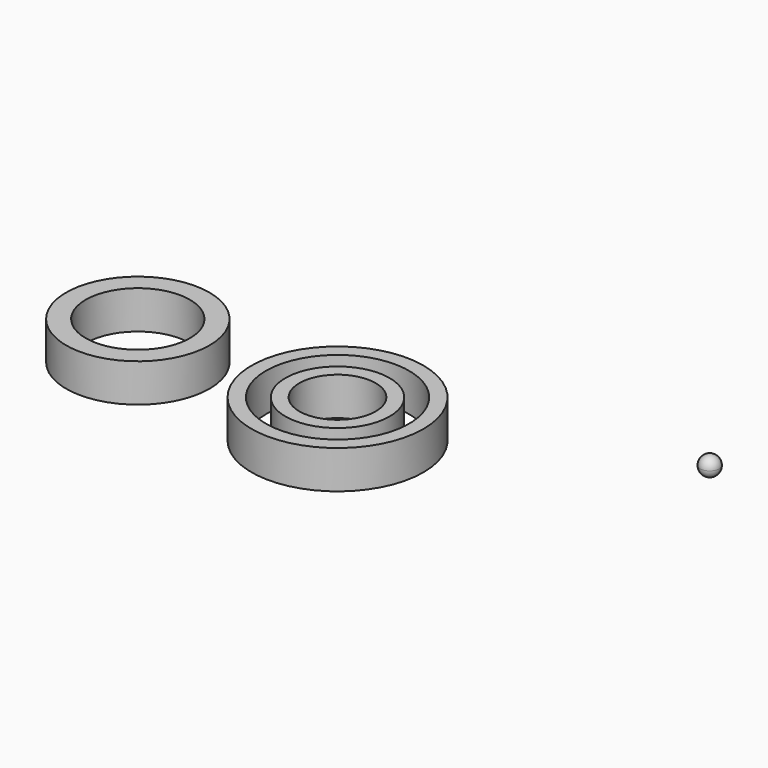
from build123d import *

# Parameters (mm, degrees)
F0_R      = 14.2875
F1_DEPTH  = 6.35
F3_D      = 23.8125
F4_R      = 8.6614
F5_DEPTH  = 6.35
F7_D      = 12.7
F8_R      = 1.5875
F9_DEPTH  = 3.175
F10_R     = 1.58749
F11_R     = 11.9126
F12_DEPTH = 6.35
F13_D     = 17.3228


# Not quite as in the source:
# - a fillet or chamfer is up to 0.001 mm smaller than in the source, because OpenCascade refuses the exact size


with BuildPart() as f1:
    # F0 (on Top) → F1 (new body)
    with BuildSketch(Plane.XY):
        with Locations((-43.9736843109, -22.3933495581)):
            Circle(F0_R)
    extrude(amount=F1_DEPTH)

    # F3 (through all)
    with Locations(Plane.XY.offset(6.35)):
        with Locations((-43.9736843109, -22.3933495581)):
            Hole(F3_D / 2)


with BuildPart() as f5:
    # F4 (on Top) → F5 (new body)
    with BuildSketch(Plane.XY):
        with Locations((-43.9736843109, -22.3933495581)):
            Circle(F4_R)
    extrude(amount=F5_DEPTH)

    # F7 (through all)
    with Locations(Plane.XY.offset(6.35)):
        with Locations((-43.9736843109, -22.3933495581)):
            Hole(F7_D / 2)


with BuildPart() as f9:
    # F8 (on Top) → F9 (new body)
    with BuildSketch(Plane.XY):
        Circle(F8_R)
    extrude(amount=F9_DEPTH)

    # F10 (radius 1.5875 in the source; OpenCascade refuses exactly that, so slightly less here)
    f10_edges = [f9.edges().sort_by_distance(p)[0] for p in [
        (-1.5875, 0, 3.175),
        (-1.5875, 0, 0),
    ]]
    fillet(f10_edges, radius=F10_R)


with BuildPart() as f12:
    # F11 (on face) → F12 (new body)
    with BuildSketch(Plane.XY.offset(6.35)):
        with Locations((-70.3552216291, -30.9257358313)):
            Circle(F11_R)
    extrude(amount=F12_DEPTH)

    # F13 (through all)
    with Locations(Plane(origin=(0, 0, 6.35), x_dir=(1, 0, 0), z_dir=(0, 0, -1))):
        with Locations((-70.3552216291, 30.9257358313)):
            Hole(F13_D / 2)


solid = Compound([f1.part, f5.part, f9.part, f12.part])
